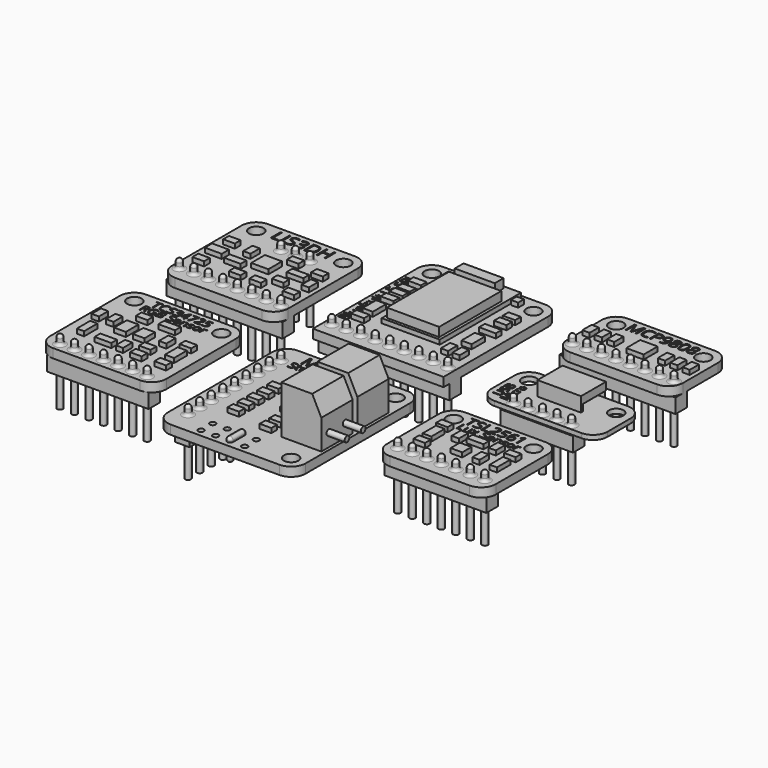
from build123d import *

# Parameters (mm, degrees)
F0_R            = 0.508
F0_R_2          = 1.27
F1_DEPTH        = 1.5875
F2_DEPTH        = 0.79375
F3_W            = 10.16
F3_H            = 17.78
F3_W_2          = 1.27
F3_H_2          = 1.27
F3_W_3          = 2.159
F3_W_4          = 2.921
F3_W_5          = 1.778
F3_H_3          = 2.921
F3_H_4          = 2.032
F3_W_6          = 2.286
F3_H_5          = 2.9464
F4_DEPTH        = 0.79375
F5_W            = 9.144
F5_H            = 13.589
F5_W_2          = 7.0104
F5_H_2          = 1.9304
F6_DEPTH        = 1.5875
F7_W            = 17.78
F7_H            = 2.54
F8_DEPTH        = 2.54
F7_W_2          = 20.32
F7_W_3          = 7.62
F7_R            = 0.508
F7_W_4          = 2.54
F7_H_2          = 22.86
F7_W_5          = 12.7
F7_W_6          = 22.86
F9_DEPTH        = 8.255
F9_DEPTH_BACK   = 3.175
F10_DEPTH       = 0.79375
F11_R           = 0.50799
F11_2_R         = 0.50799
F11_3_R         = 0.50799
F11_4_R         = 0.50799
F11_5_R         = 0.50799
F11_6_R         = 0.50799
F11_7_R         = 0.50799
F13_DEPTH       = 0.762
F13_DEPTH_BACK  = 1.5875
F14_DEPTH       = 1.5875
F15_W           = 6.985
F15_H           = 6.858
F15_R           = 0.508
F16_DEPTH       = 8.382
F17_SIZE2       = 1.5875
F17_SIZE        = 3.175
F18_SIZE2       = 1.5875
F18_SIZE        = 3.175
F19_R           = 0.508
F20_DEPTH       = 3.175
F21_DEPTH       = 1.5875
F21_DEPTH_BACK  = 6.35
F22_R           = 0.50799
F23_W           = 1.27
F23_H           = 2.032
F23_W_2         = 2.032
F23_H_2         = 1.27
F23_W_3         = 2.921
F23_H_3         = 2.921
F24_DEPTH       = 0.79375
F23_W_4         = 7.62
F23_H_4         = 5.4864
F23_W_5         = 2.9464
F23_H_5         = 1.5875
F23_W_6         = 2.9972
F23_H_6         = 2.9972
F23_H_7         = 2.794
F23_H_8         = 2.286
F23_W_7         = 1.5875
F23_W_8         = 1.524
F23_W_9         = 3.048
F23_H_9         = 3.048
F25_DEPTH       = 0.79375
F25_DEPTH_BACK  = 1.74625
F27_DEPTH       = 5.08
F28_TEXT_SIZE   = 3.0305741984
F28_TEXT_SIZE_2 = 2.2091458857
F28_TEXT_SIZE_3 = 2.0715317305
F28_TEXT_SIZE_4 = 2.8646616541
F28_TEXT_SIZE_5 = 2.091610911
F28_TEXT_SIZE_6 = 2.1665037761
F28_TEXT_SIZE_7 = 2.5736521957
F28_TEXT_SIZE_8 = 2.083851119
F28_TEXT_SIZE_9 = 2.7485575399
F29_DEPTH       = 0.254
F30_TEXT_SIZE   = 1.9694693482
F30_TEXT_SIZE_2 = 1.7952644599
F31_DEPTH       = 0.254


# Not quite as in the source:
# - a fillet or chamfer is up to 0.001 mm smaller than in the source, because OpenCascade refuses the exact size
# - Text() gives the source's letters only with a copy of the font that has no kerning and outlines rounded to 1/6400 em; it was checked with that copy


with BuildPart() as f1:
    # F0 (on Top) → F1 (new body)
    with BuildSketch(Plane.XY):
        with BuildLine():
            Line((0, 22.86), (0, 0))
            Line((0, 0), (22.86, 0))
            Line((22.86, 0), (22.86, 22.86))
            ThreePointArc((22.86, 22.86), (22.1160512242, 24.6560512242), (20.32, 25.4))
            Line((20.32, 25.4), (2.54, 25.4))
            ThreePointArc((2.54, 25.4), (0.7439487758, 24.6560512242), (0, 22.86))
        make_face()
        with Locations((1.27, 2.54)):
            Circle(F0_R, mode=Mode.SUBTRACT)
        with Locations((3.81, 2.54)):
            Circle(F0_R, mode=Mode.SUBTRACT)
        with Locations((6.35, 2.54)):
            Circle(F0_R, mode=Mode.SUBTRACT)
        with Locations((8.89, 2.54)):
            Circle(F0_R, mode=Mode.SUBTRACT)
        with Locations((2.54, 22.86)):
            Circle(F0_R_2, mode=Mode.SUBTRACT)
        with Locations((11.43, 2.54)):
            Circle(F0_R, mode=Mode.SUBTRACT)
        with Locations((13.97, 2.54)):
            Circle(F0_R, mode=Mode.SUBTRACT)
        with Locations((16.51, 2.54)):
            Circle(F0_R, mode=Mode.SUBTRACT)
        with Locations((19.05, 2.54)):
            Circle(F0_R, mode=Mode.SUBTRACT)
        with Locations((21.59, 2.54)):
            Circle(F0_R, mode=Mode.SUBTRACT)
        with Locations((20.32, 22.86)):
            Circle(F0_R_2, mode=Mode.SUBTRACT)
    extrude(amount=F1_DEPTH)

    # F3 (on face) → F4 (join)
    with BuildSketch(Plane.XY.offset(1.5875)):
        with Locations((11.43, 16.002)):
            Rectangle(F3_W, F3_H)
        with Locations((5.461, 22.987)):
            Rectangle(F3_W_2, F3_H_2)
        with Locations((17.399, 22.987)):
            Rectangle(F3_W_2, F3_H_2)
        with Locations((19.8755, 18.669)):
            Rectangle(F3_W_3, F3_H_2)
        with Locations((19.8755, 16.764)):
            Rectangle(F3_W_3, F3_H_2)
        with Locations((19.8755, 13.97)):
            Rectangle(F3_W_4, F3_H_2)
        with Locations((19.8755, 10.2235)):
            Rectangle(F3_W_5, F3_H_3)
        with Locations((20.8915, 6.223)):
            Rectangle(F3_W_2, F3_H_4)
        with Locations((18.8595, 6.223)):
            Rectangle(F3_W_2, F3_H_4)
        with Locations((3.3274, 6.223)):
            Rectangle(F3_W_6, F3_H_2)
        with Locations((3.3274, 9.2964)):
            Rectangle(F3_W_5, F3_H_5)
        with Locations((3.3274, 12.7)):
            Rectangle(F3_W_6, F3_H_2)
        with Locations((3.3274, 18.669)):
            Rectangle(F3_W_6, F3_H_2)
        with Locations((3.3274, 16.256)):
            Rectangle(F3_W_6, F3_H_2)
        with Locations((3.3274, 14.605)):
            Rectangle(F3_W_6, F3_H_2)
    extrude(amount=F4_DEPTH)

    # F5 (on face) → F6 (join)
    with BuildSketch(Plane.XY.offset(2.38125)):
        with Locations((11.43, 14.4145)):
            Rectangle(F5_W, F5_H)
        with Locations((10.3632, 23.4188)):
            Rectangle(F5_W_2, F5_H_2)
    extrude(amount=F6_DEPTH)

    # F7 (on face) → F8, piece 5 (join)
    with BuildSketch(Plane(origin=(0, 0, 0), x_dir=(1, 0, 0), z_dir=(0, 0, -1))):
        with Locations((11.43, -2.54)):
            Rectangle(F7_W_6, F7_H)
        with Locations((1.27, -2.54)):
            Circle(F7_R, mode=Mode.SUBTRACT)
        with Locations((3.81, -2.54)):
            Circle(F7_R, mode=Mode.SUBTRACT)
        with Locations((6.35, -2.54)):
            Circle(F7_R, mode=Mode.SUBTRACT)
        with Locations((8.89, -2.54)):
            Circle(F7_R, mode=Mode.SUBTRACT)
        with Locations((11.43, -2.54)):
            Circle(F7_R, mode=Mode.SUBTRACT)
        with Locations((13.97, -2.54)):
            Circle(F7_R, mode=Mode.SUBTRACT)
        with Locations((16.51, -2.54)):
            Circle(F7_R, mode=Mode.SUBTRACT)
        with Locations((19.05, -2.54)):
            Circle(F7_R, mode=Mode.SUBTRACT)
        with Locations((21.59, -2.54)):
            Circle(F7_R, mode=Mode.SUBTRACT)
    extrude(amount=F8_DEPTH)

    # F0 (on Top) → F9 (join, two sides)
    with BuildSketch(Plane.XY) as f9_sk:
        with Locations((1.27, 2.54)):
            Circle(F0_R)
        with Locations((3.81, 2.54)):
            Circle(F0_R)
        with Locations((6.35, 2.54)):
            Circle(F0_R)
        with Locations((8.89, 2.54)):
            Circle(F0_R)
        with Locations((11.43, 2.54)):
            Circle(F0_R)
        with Locations((13.97, 2.54)):
            Circle(F0_R)
        with Locations((16.51, 2.54)):
            Circle(F0_R)
        with Locations((19.05, 2.54)):
            Circle(F0_R)
        with Locations((21.59, 2.54)):
            Circle(F0_R)
    extrude(amount=-F9_DEPTH)
    extrude(f9_sk.sketch, amount=F9_DEPTH_BACK)

    # F11 (radius 0.508 in the source; OpenCascade refuses exactly that, so slightly less here)
    f11_edges = [f1.edges().sort_by_distance(p)[0] for p in [
        (0.762, 2.54, 1.5875),
        (1.778, 2.54, 2.38125),
        (0.762, 2.54, 3.175),
        (3.302, 2.54, 1.5875),
        (4.318, 2.54, 2.38125),
        (3.302, 2.54, 3.175),
        (5.842, 2.54, 1.5875),
        (6.858, 2.54, 2.38125),
        (5.842, 2.54, 3.175),
        (8.382, 2.54, 1.5875),
        (9.398, 2.54, 2.38125),
        (8.382, 2.54, 3.175),
        (10.922, 2.54, 1.5875),
        (11.938, 2.54, 2.38125),
        (10.922, 2.54, 3.175),
        (13.462, 2.54, 1.5875),
        (14.478, 2.54, 2.38125),
        (13.462, 2.54, 3.175),
        (16.002, 2.54, 1.5875),
        (17.018, 2.54, 2.38125),
        (16.002, 2.54, 3.175),
        (18.542, 2.54, 1.5875),
        (19.558, 2.54, 2.38125),
        (18.542, 2.54, 3.175),
        (21.082, 2.54, 1.5875),
        (22.098, 2.54, 2.38125),
        (21.082, 2.54, 3.175),
    ]]
    fillet(f11_edges, radius=F11_R)


with BuildPart() as f1b:
    # F0 (on Top) → F1, piece 2 (new body)
    with BuildSketch(Plane.XY):
        with BuildLine():
            Line((-24.13, 0), (-8.89, 0))
            ThreePointArc((-8.89, 0), (-7.0939487758, 0.7439487758), (-6.35, 2.54))
            Line((-6.35, 2.54), (-6.35, 17.78))
            ThreePointArc((-6.35, 17.78), (-7.0939487758, 19.5760512242), (-8.89, 20.32))
            Line((-8.89, 20.32), (-24.13, 20.32))
            ThreePointArc((-24.13, 20.32), (-25.9260512242, 19.5760512242), (-26.67, 17.78))
            Line((-26.67, 17.78), (-26.67, 2.54))
            ThreePointArc((-26.67, 2.54), (-25.9260512242, 0.7439487758), (-24.13, 0))
        make_face()
        with Locations((-25.4, 2.54)):
            Circle(F0_R, mode=Mode.SUBTRACT)
        with Locations((-22.86, 2.54)):
            Circle(F0_R, mode=Mode.SUBTRACT)
        with Locations((-20.32, 2.54)):
            Circle(F0_R, mode=Mode.SUBTRACT)
        with Locations((-17.78, 2.54)):
            Circle(F0_R, mode=Mode.SUBTRACT)
        with Locations((-15.24, 2.54)):
            Circle(F0_R, mode=Mode.SUBTRACT)
        with Locations((-12.7, 2.54)):
            Circle(F0_R, mode=Mode.SUBTRACT)
        with Locations((-10.16, 2.54)):
            Circle(F0_R, mode=Mode.SUBTRACT)
        with Locations((-7.62, 2.54)):
            Circle(F0_R, mode=Mode.SUBTRACT)
        with Locations((-17.78, 15.24)):
            Circle(F0_R, mode=Mode.SUBTRACT)
        with Locations((-24.13, 17.78)):
            Circle(F0_R_2, mode=Mode.SUBTRACT)
        with Locations((-15.24, 15.24)):
            Circle(F0_R, mode=Mode.SUBTRACT)
        with Locations((-12.7, 15.24)):
            Circle(F0_R, mode=Mode.SUBTRACT)
        with Locations((-8.89, 17.78)):
            Circle(F0_R_2, mode=Mode.SUBTRACT)
    extrude(amount=F1_DEPTH)

    # F7 (on face) → F8, piece 2 (join)
    with BuildSketch(Plane(origin=(0, 0, 0), x_dir=(1, 0, 0), z_dir=(0, 0, -1))):
        with Locations((-16.51, -2.54)):
            Rectangle(F7_W_2, F7_H)
        with Locations((-15.24, -15.24)):
            Rectangle(F7_W_3, F7_H)
        with Locations((-15.24, -15.24)):
            Circle(F7_R, mode=Mode.SUBTRACT)
        with Locations((-15.24, -15.24)):
            Circle(F7_R)
    extrude(amount=F8_DEPTH)

    # F0 (on Top) → F9, piece 2 (join, two sides)
    with BuildSketch(Plane.XY) as f9_2_sk:
        with Locations((-25.4, 2.54)):
            Circle(F0_R)
        with Locations((-22.86, 2.54)):
            Circle(F0_R)
        with Locations((-20.32, 2.54)):
            Circle(F0_R)
        with Locations((-17.78, 2.54)):
            Circle(F0_R)
        with Locations((-15.24, 2.54)):
            Circle(F0_R)
        with Locations((-12.7, 2.54)):
            Circle(F0_R)
        with Locations((-10.16, 2.54)):
            Circle(F0_R)
        with Locations((-7.62, 2.54)):
            Circle(F0_R)
        with Locations((-12.7, 15.24)):
            Circle(F0_R)
        with Locations((-15.24, 15.24)):
            Circle(F0_R)
        with Locations((-17.78, 15.24)):
            Circle(F0_R)
    extrude(amount=-F9_DEPTH)
    extrude(f9_2_sk.sketch, amount=F9_DEPTH_BACK)

    # F11#2 (radius 0.508 in the source; OpenCascade refuses exactly that, so slightly less here)
    f11_2_edges = [f1b.edges().sort_by_distance(p)[0] for p in [
        (-25.908, 2.54, 1.5875),
        (-24.892, 2.54, 2.38125),
        (-25.908, 2.54, 3.175),
        (-23.368, 2.54, 1.5875),
        (-22.352, 2.54, 2.38125),
        (-23.368, 2.54, 3.175),
        (-18.288, 2.54, 1.5875),
        (-17.272, 2.54, 2.38125),
        (-18.288, 2.54, 3.175),
        (-20.828, 2.54, 1.5875),
        (-19.812, 2.54, 2.38125),
        (-20.828, 2.54, 3.175),
        (-15.748, 2.54, 1.5875),
        (-14.732, 2.54, 2.38125),
        (-15.748, 2.54, 3.175),
        (-13.208, 2.54, 1.5875),
        (-12.192, 2.54, 2.38125),
        (-13.208, 2.54, 3.175),
        (-10.668, 2.54, 1.5875),
        (-9.652, 2.54, 2.38125),
        (-10.668, 2.54, 3.175),
        (-8.128, 2.54, 1.5875),
        (-7.112, 2.54, 2.38125),
        (-8.128, 2.54, 3.175),
        (-13.208, 15.24, 1.5875),
        (-12.192, 15.24, 2.38125),
        (-13.208, 15.24, 3.175),
        (-15.748, 15.24, 1.5875),
        (-14.732, 15.24, 2.38125),
        (-15.748, 15.24, 3.175),
        (-18.288, 15.24, 1.5875),
        (-17.272, 15.24, 2.38125),
        (-18.288, 15.24, 3.175),
    ]]
    fillet(f11_2_edges, radius=F11_2_R)

    # F23 (on face) → F24, piece 3 (join)
    with BuildSketch(Plane.XY.offset(1.5875)):
        with Locations((-24.0792, 9.11225)):
            Rectangle(F23_W_5, F23_H_5)
        with Locations((-24.13, 12.446)):
            Rectangle(F23_W_2, F23_H_2)
        with Locations((-20.193, 11.811)):
            Rectangle(F23_W, F23_H)
        with Locations((-20.193, 8.255)):
            Rectangle(F23_W_3, F23_H_2)
        with Locations((-16.2814, 10.2362)):
            Rectangle(F23_W_6, F23_H_6)
        with Locations((-13.589, 13.208)):
            Rectangle(F23_W_2, F23_H_2)
        with Locations((-10.8585, 10.287)):
            Rectangle(F23_W_3, F23_H_2)
        with Locations((-11.684, 7.5184)):
            Rectangle(F23_W_2, F23_H_2)
        with Locations((-7.747, 9.017)):
            Rectangle(F23_W, F23_H)
        with Locations((-8.636, 12.319)):
            Rectangle(F23_W_2, F23_H_2)
        with Locations((-8.255, 5.588)):
            Rectangle(F23_W_2, F23_H_2)
        with Locations((-14.0716, 5.588)):
            Rectangle(F23_W_2, F23_H_2)
        with Locations((-17.653, 5.588)):
            Rectangle(F23_W_2, F23_H_2)
        with Locations((-24.13, 5.715)):
            Rectangle(F23_W_2, F23_H_2)
    extrude(amount=F24_DEPTH)


with BuildPart() as f1c:
    # F0 (on Top) → F1, piece 3 (new body)
    with BuildSketch(Plane.XY):
        with BuildLine():
            ThreePointArc((-6.35, -8.89), (-7.0939487758, -7.0939487758), (-8.89, -6.35))
            Line((-8.89, -6.35), (-24.13, -6.35))
            ThreePointArc((-24.13, -6.35), (-25.9260512242, -7.0939487758), (-26.67, -8.89))
            Line((-26.67, -8.89), (-26.67, -24.13))
            ThreePointArc((-26.67, -24.13), (-25.9260512242, -25.9260512242), (-24.13, -26.67))
            Line((-24.13, -26.67), (-8.89, -26.67))
            ThreePointArc((-8.89, -26.67), (-7.0939487758, -25.9260512242), (-6.35, -24.13))
            Line((-6.35, -24.13), (-6.35, -8.89))
        make_face()
        with Locations((-24.13, -25.146)):
            Circle(F0_R, mode=Mode.SUBTRACT)
        with Locations((-21.59, -25.146)):
            Circle(F0_R, mode=Mode.SUBTRACT)
        with Locations((-19.05, -25.146)):
            Circle(F0_R, mode=Mode.SUBTRACT)
        with Locations((-16.51, -25.146)):
            Circle(F0_R, mode=Mode.SUBTRACT)
        with Locations((-13.97, -25.146)):
            Circle(F0_R, mode=Mode.SUBTRACT)
        with Locations((-11.43, -25.146)):
            Circle(F0_R, mode=Mode.SUBTRACT)
        with Locations((-8.89, -25.146)):
            Circle(F0_R, mode=Mode.SUBTRACT)
        with Locations((-24.13, -8.89)):
            Circle(F0_R_2, mode=Mode.SUBTRACT)
        with Locations((-8.89, -8.89)):
            Circle(F0_R_2, mode=Mode.SUBTRACT)
    extrude(amount=F1_DEPTH)

    # F7 (on face) → F8 (join)
    with BuildSketch(Plane(origin=(0, 0, 0), x_dir=(1, 0, 0), z_dir=(0, 0, -1))):
        with Locations((-16.51, 25.146)):
            Rectangle(F7_W, F7_H)
    extrude(amount=F8_DEPTH)

    # F0 (on Top) → F9, piece 3 (join, two sides)
    with BuildSketch(Plane.XY) as f9_3_sk:
        with Locations((-24.13, -25.146)):
            Circle(F0_R)
        with Locations((-21.59, -25.146)):
            Circle(F0_R)
        with Locations((-19.05, -25.146)):
            Circle(F0_R)
        with Locations((-16.51, -25.146)):
            Circle(F0_R)
        with Locations((-13.97, -25.146)):
            Circle(F0_R)
        with Locations((-11.43, -25.146)):
            Circle(F0_R)
        with Locations((-8.89, -25.146)):
            Circle(F0_R)
    extrude(amount=-F9_DEPTH)
    extrude(f9_3_sk.sketch, amount=F9_DEPTH_BACK)

    # F11#3 (radius 0.508 in the source; OpenCascade refuses exactly that, so slightly less here)
    f11_3_edges = [f1c.edges().sort_by_distance(p)[0] for p in [
        (-9.398, -25.146, 1.5875),
        (-8.382, -25.146, 2.38125),
        (-9.398, -25.146, 3.175),
        (-11.938, -25.146, 1.5875),
        (-10.922, -25.146, 2.38125),
        (-11.938, -25.146, 3.175),
        (-14.478, -25.146, 1.5875),
        (-13.462, -25.146, 2.38125),
        (-14.478, -25.146, 3.175),
        (-17.018, -25.146, 1.5875),
        (-16.002, -25.146, 2.38125),
        (-17.018, -25.146, 3.175),
        (-19.558, -25.146, 1.5875),
        (-18.542, -25.146, 2.38125),
        (-19.558, -25.146, 3.175),
        (-22.098, -25.146, 1.5875),
        (-21.082, -25.146, 2.38125),
        (-22.098, -25.146, 3.175),
        (-24.638, -25.146, 1.5875),
        (-23.622, -25.146, 2.38125),
        (-24.638, -25.146, 3.175),
    ]]
    fillet(f11_3_edges, radius=F11_3_R)

    # F23 (on face) → F24, piece 4 (join)
    with BuildSketch(Plane.XY.offset(1.5875)):
        with Locations((-24.765, -15.621)):
            Rectangle(F23_W, F23_H)
        with Locations((-22.225, -15.621)):
            Rectangle(F23_W, F23_H)
        with Locations((-19.304, -12.7)):
            Rectangle(F23_W_2, F23_H_2)
        with Locations((-19.431, -16.51)):
            Rectangle(F23_W_2, F23_H_7)
        with Locations((-16.256, -16.637)):
            Rectangle(F23_W_2, F23_H_8)
        with Locations((-14.9225, -12.7)):
            Rectangle(F23_W_3, F23_H_2)
        with Locations((-12.573, -16.129)):
            Rectangle(F23_W, F23_H)
        with Locations((-9.398, -15.494)):
            Rectangle(F23_W_2, F23_H_2)
        with Locations((-9.23925, -18.415)):
            Rectangle(F23_W_7, F23_H_7)
        with Locations((-13.208, -21.59)):
            Rectangle(F23_W_2, F23_H_2)
        with Locations((-13.462, -19.304)):
            Rectangle(F23_W_2, F23_H_2)
        with Locations((-16.383, -20.828)):
            Rectangle(F23_W, F23_H)
        with Locations((-19.3675, -21.082)):
            Rectangle(F23_W_3, F23_H_2)
        with Locations((-23.622, -19.8501)):
            Rectangle(F23_W, F23_H_3)
        with Locations((-8.9408, -21.59)):
            Rectangle(F23_W_2, F23_H_2)
    extrude(amount=F24_DEPTH)


with BuildPart() as f1d:
    # F0 (on Top) → F1, piece 4 (new body)
    with BuildSketch(Plane.XY):
        with BuildLine():
            Line((21.59, -6.35), (2.54, -6.35))
            ThreePointArc((2.54, -6.35), (0.7439487758, -7.0939487758), (0, -8.89))
            Line((0, -8.89), (0, -31.75))
            ThreePointArc((0, -31.75), (0.7439487758, -33.5460512242), (2.54, -34.29))
            Line((2.54, -34.29), (21.59, -34.29))
            ThreePointArc((21.59, -34.29), (23.3860512242, -33.5460512242), (24.13, -31.75))
            Line((24.13, -31.75), (24.13, -8.89))
            ThreePointArc((24.13, -8.89), (23.3860512242, -7.0939487758), (21.59, -6.35))
        make_face()
        with Locations((2.54, -30.48)):
            Circle(F0_R, mode=Mode.SUBTRACT)
        with Locations((6.858, -33.02)):
            Circle(F0_R, mode=Mode.SUBTRACT)
        with Locations((9.398, -33.02)):
            Circle(F0_R, mode=Mode.SUBTRACT)
        with Locations((6.858, -30.48)):
            Circle(F0_R, mode=Mode.SUBTRACT)
        with Locations((9.398, -30.48)):
            Circle(F0_R, mode=Mode.SUBTRACT)
        with Locations((2.54, -27.94)):
            Circle(F0_R, mode=Mode.SUBTRACT)
        with Locations((2.54, -25.4)):
            Circle(F0_R, mode=Mode.SUBTRACT)
        with Locations((2.54, -22.86)):
            Circle(F0_R, mode=Mode.SUBTRACT)
        with Locations((2.54, -20.32)):
            Circle(F0_R, mode=Mode.SUBTRACT)
        with Locations((2.54, -17.78)):
            Circle(F0_R, mode=Mode.SUBTRACT)
        with Locations((2.54, -15.24)):
            Circle(F0_R, mode=Mode.SUBTRACT)
        with Locations((2.54, -12.7)):
            Circle(F0_R, mode=Mode.SUBTRACT)
        with Locations((2.54, -10.16)):
            Circle(F0_R, mode=Mode.SUBTRACT)
        with Locations((11.938, -33.02)):
            Circle(F0_R, mode=Mode.SUBTRACT)
        with Locations((14.478, -33.02)):
            Circle(F0_R, mode=Mode.SUBTRACT)
        with Locations((11.938, -30.48)):
            Circle(F0_R, mode=Mode.SUBTRACT)
        with Locations((14.478, -30.48)):
            Circle(F0_R, mode=Mode.SUBTRACT)
        with Locations((21.59, -31.75)):
            Circle(F0_R_2, mode=Mode.SUBTRACT)
        with Locations((20.066, -26.035)):
            Circle(F0_R, mode=Mode.SUBTRACT)
        with Locations((20.066, -22.479)):
            Circle(F0_R, mode=Mode.SUBTRACT)
        with Locations((20.066, -18.161)):
            Circle(F0_R, mode=Mode.SUBTRACT)
        with Locations((20.066, -14.605)):
            Circle(F0_R, mode=Mode.SUBTRACT)
        with Locations((21.59, -8.89)):
            Circle(F0_R_2, mode=Mode.SUBTRACT)
    extrude(amount=F1_DEPTH)

    # F7 (on face) → F8, piece 3 (join)
    with BuildSketch(Plane(origin=(0, 0, 0), x_dir=(1, 0, 0), z_dir=(0, 0, -1))):
        with Locations((2.54, 20.32)):
            Rectangle(F7_W_4, F7_H_2)
    extrude(amount=F8_DEPTH)

    # F0 (on Top) → F9, piece 4 (join, two sides)
    with BuildSketch(Plane.XY) as f9_4_sk:
        with Locations((2.54, -30.48)):
            Circle(F0_R)
        with Locations((2.54, -27.94)):
            Circle(F0_R)
        with Locations((2.54, -25.4)):
            Circle(F0_R)
        with Locations((2.54, -22.86)):
            Circle(F0_R)
        with Locations((2.54, -20.32)):
            Circle(F0_R)
        with Locations((2.54, -17.78)):
            Circle(F0_R)
        with Locations((2.54, -15.24)):
            Circle(F0_R)
        with Locations((2.54, -12.7)):
            Circle(F0_R)
        with Locations((2.54, -10.16)):
            Circle(F0_R)
    extrude(amount=-F9_DEPTH)
    extrude(f9_4_sk.sketch, amount=F9_DEPTH_BACK)

    # F11#4 (radius 0.508 in the source; OpenCascade refuses exactly that, so slightly less here)
    f11_4_edges = [f1d.edges().sort_by_distance(p)[0] for p in [
        (2.032, -17.78, 1.5875),
        (3.048, -17.78, 2.38125),
        (2.032, -17.78, 3.175),
        (2.032, -15.24, 1.5875),
        (3.048, -15.24, 2.38125),
        (2.032, -15.24, 3.175),
        (2.032, -12.7, 1.5875),
        (3.048, -12.7, 2.38125),
        (2.032, -12.7, 3.175),
        (2.032, -10.16, 1.5875),
        (3.048, -10.16, 2.38125),
        (2.032, -10.16, 3.175),
        (2.032, -20.32, 1.5875),
        (3.048, -20.32, 2.38125),
        (2.032, -20.32, 3.175),
        (2.032, -22.86, 1.5875),
        (3.048, -22.86, 2.38125),
        (2.032, -22.86, 3.175),
        (2.032, -25.4, 1.5875),
        (3.048, -25.4, 2.38125),
        (2.032, -25.4, 3.175),
        (2.032, -27.94, 1.5875),
        (3.048, -27.94, 2.38125),
        (2.032, -27.94, 3.175),
        (2.032, -30.48, 1.5875),
        (3.048, -30.48, 2.38125),
        (2.032, -30.48, 3.175),
    ]]
    fillet(f11_4_edges, radius=F11_4_R)

    # F12 (on face) → F13 (join, two sides)
    with BuildSketch(Plane.XY.offset(1.5875)) as f13_sk:
        with BuildLine():
            ThreePointArc((12.446, -30.48), (11.938, -30.988), (11.43, -30.48))
            Line((11.43, -30.48), (11.43, -33.02))
            ThreePointArc((11.43, -33.02), (11.938, -32.512), (12.446, -33.02))
            Line((12.446, -33.02), (12.446, -30.48))
        make_face()
        with BuildLine():
            ThreePointArc((12.446, -30.48), (11.938, -29.972), (11.43, -30.48))
            ThreePointArc((11.43, -30.48), (11.938, -30.988), (12.446, -30.48))
        make_face()
        with BuildLine():
            ThreePointArc((12.446, -33.02), (11.938, -32.512), (11.43, -33.02))
            ThreePointArc((11.43, -33.02), (11.938, -33.528), (12.446, -33.02))
        make_face()
    extrude(amount=F13_DEPTH)
    extrude(f13_sk.sketch, amount=-F13_DEPTH_BACK)

    # F0 (on Top) → F14 (join)
    with BuildSketch(Plane.XY):
        with Locations((11.938, -33.02)):
            Circle(F0_R)
        with Locations((11.938, -30.48)):
            Circle(F0_R)
    extrude(amount=-F14_DEPTH)

    # F15 (on face) → F16 (join)
    with BuildSketch(Plane.XY.offset(1.5875)):
        with Locations((20.1295, -16.383)):
            Rectangle(F15_W, F15_H)
        with Locations((20.066, -18.161)):
            Circle(F15_R, mode=Mode.SUBTRACT)
        with Locations((20.066, -14.605)):
            Circle(F15_R, mode=Mode.SUBTRACT)
        with Locations((20.1295, -24.257)):
            Rectangle(F15_W, F15_H)
        with Locations((20.066, -26.035)):
            Circle(F15_R, mode=Mode.SUBTRACT)
        with Locations((20.066, -22.479)):
            Circle(F15_R, mode=Mode.SUBTRACT)
        with Locations((20.066, -26.035)):
            Circle(F15_R)
        with Locations((20.066, -22.479)):
            Circle(F15_R)
        with Locations((20.066, -14.605)):
            Circle(F15_R)
        with Locations((20.066, -18.161)):
            Circle(F15_R)
    extrude(amount=F16_DEPTH)

    # F17
    f17_edges = [f1d.edges().sort_by_distance(p)[0] for p in [
        (23.622, -24.257, 9.9695),
    ]]
    f17_side = f1d.faces().sort_by_distance((23.622, -24.257, 5.7785))[0]
    chamfer(f17_edges, length=F17_SIZE, length2=F17_SIZE2, reference=f17_side)

    # F18
    f18_edges = [f1d.edges().sort_by_distance(p)[0] for p in [
        (23.622, -16.383, 9.9695),
    ]]
    f18_side = f1d.faces().sort_by_distance((23.622, -16.383, 5.7785))[0]
    chamfer(f18_edges, length=F18_SIZE, length2=F18_SIZE2, reference=f18_side)

    # F19 (on face) → F20 (join)
    with BuildSketch(Plane.YZ.offset(23.622)):
        with Locations((-26.035, 3.8735)):
            Circle(F19_R)
        with Locations((-22.479, 3.8735)):
            Circle(F19_R)
    extrude(amount=F20_DEPTH)

    # F0 (on Top) → F21 (join, two sides)
    with BuildSketch(Plane.XY) as f21_sk:
        with Locations((20.066, -26.035)):
            Circle(F0_R)
        with Locations((20.066, -22.479)):
            Circle(F0_R)
    extrude(amount=-F21_DEPTH)
    extrude(f21_sk.sketch, amount=F21_DEPTH_BACK)

    # F22 (radius 0.508 in the source; OpenCascade refuses exactly that, so slightly less here)
    f22_edges = [f1d.edges().sort_by_distance(p)[0] for p in [
        (12.446, -33.02, -0.79375),
        (11.43, -33.02, 0),
        (11.43, -33.02, -1.5875),
        (12.446, -30.48, -0.79375),
        (11.43, -30.48, 0),
        (11.43, -30.48, -1.5875),
        (20.574, -22.479, -0.79375),
        (19.558, -22.479, 0),
        (19.558, -22.479, -1.5875),
        (20.574, -26.035, -0.79375),
        (19.558, -26.035, 0),
        (19.558, -26.035, -1.5875),
        (11.43, -31.75, 2.3495),
        (11.938, -33.528, 2.3495),
        (12.446, -31.75, 2.3495),
        (11.938, -29.972, 2.3495),
    ]]
    fillet(f22_edges, radius=F22_R)

    # F23 (on face) → F24 (join)
    with BuildSketch(Plane.XY.offset(1.5875)):
        with Locations((8.5598, -14.605)):
            Rectangle(F23_W, F23_H)
        with Locations((7.3914, -17.399)):
            Rectangle(F23_W_2, F23_H_2)
        with Locations((7.3914, -19.558)):
            Rectangle(F23_W_2, F23_H_2)
        with Locations((7.3914, -21.717)):
            Rectangle(F23_W_2, F23_H_2)
        with Locations((7.3914, -23.876)):
            Rectangle(F23_W_2, F23_H_2)
        with Locations((7.3914, -26.035)):
            Rectangle(F23_W_2, F23_H_2)
        with Locations((13.2969, -20.5105)):
            Rectangle(F23_W_3, F23_H_3)
        with Locations((13.8684, -24.9936)):
            Rectangle(F23_W_2, F23_H_2)
        with Locations((13.8684, -27.0637)):
            Rectangle(F23_W_2, F23_H_2)
        with Locations((12.065, -15.494)):
            Rectangle(F23_W, F23_H)
        with Locations((14.2494, -15.494)):
            Rectangle(F23_W, F23_H)
    extrude(amount=F24_DEPTH)


with BuildPart() as f1e:
    # F0 (on Top) → F1, piece 5 (new body)
    with BuildSketch(Plane.XY):
        with BuildLine():
            Line((45.72, -6.35), (31.75, -6.35))
            ThreePointArc((31.75, -6.35), (29.9539487758, -7.0939487758), (29.21, -8.89))
            Line((29.21, -8.89), (29.21, -20.32))
            ThreePointArc((29.21, -20.32), (29.9539487758, -22.1160512242), (31.75, -22.86))
            Line((31.75, -22.86), (45.72, -22.86))
            ThreePointArc((45.72, -22.86), (47.5160512242, -22.1160512242), (48.26, -20.32))
            Line((48.26, -20.32), (48.26, -8.89))
            ThreePointArc((48.26, -8.89), (47.5160512242, -7.0939487758), (45.72, -6.35))
        make_face()
        with Locations((31.115, -20.32)):
            Circle(F0_R, mode=Mode.SUBTRACT)
        with Locations((33.655, -20.32)):
            Circle(F0_R, mode=Mode.SUBTRACT)
        with Locations((36.195, -20.32)):
            Circle(F0_R, mode=Mode.SUBTRACT)
        with Locations((38.735, -20.32)):
            Circle(F0_R, mode=Mode.SUBTRACT)
        with Locations((41.275, -20.32)):
            Circle(F0_R, mode=Mode.SUBTRACT)
        with Locations((43.815, -20.32)):
            Circle(F0_R, mode=Mode.SUBTRACT)
        with Locations((46.355, -20.32)):
            Circle(F0_R, mode=Mode.SUBTRACT)
        with Locations((31.75, -8.89)):
            Circle(F0_R_2, mode=Mode.SUBTRACT)
        with Locations((45.72, -8.89)):
            Circle(F0_R_2, mode=Mode.SUBTRACT)
    extrude(amount=F1_DEPTH)

    # F7 (on face) → F8, piece 6 (join)
    with BuildSketch(Plane(origin=(0, 0, 0), x_dir=(1, 0, 0), z_dir=(0, 0, -1))):
        with Locations((38.735, 20.32)):
            Rectangle(F7_W, F7_H)
    extrude(amount=F8_DEPTH)

    # F0 (on Top) → F9, piece 6 (join, two sides)
    with BuildSketch(Plane.XY) as f9_6_sk:
        with Locations((46.355, -20.32)):
            Circle(F0_R)
        with Locations((43.815, -20.32)):
            Circle(F0_R)
        with Locations((41.275, -20.32)):
            Circle(F0_R)
        with Locations((38.735, -20.32)):
            Circle(F0_R)
        with Locations((36.195, -20.32)):
            Circle(F0_R)
        with Locations((33.655, -20.32)):
            Circle(F0_R)
        with Locations((31.115, -20.32)):
            Circle(F0_R)
    extrude(amount=-F9_DEPTH)
    extrude(f9_6_sk.sketch, amount=F9_DEPTH_BACK)

    # F11#5 (radius 0.508 in the source; OpenCascade refuses exactly that, so slightly less here)
    f11_5_edges = [f1e.edges().sort_by_distance(p)[0] for p in [
        (38.227, -20.32, 1.5875),
        (39.243, -20.32, 2.38125),
        (38.227, -20.32, 3.175),
        (35.687, -20.32, 1.5875),
        (36.703, -20.32, 2.38125),
        (35.687, -20.32, 3.175),
        (33.147, -20.32, 1.5875),
        (34.163, -20.32, 2.38125),
        (33.147, -20.32, 3.175),
        (40.767, -20.32, 1.5875),
        (41.783, -20.32, 2.38125),
        (40.767, -20.32, 3.175),
        (43.307, -20.32, 1.5875),
        (44.323, -20.32, 2.38125),
        (43.307, -20.32, 3.175),
        (45.847, -20.32, 1.5875),
        (46.863, -20.32, 2.38125),
        (45.847, -20.32, 3.175),
        (30.607, -20.32, 1.5875),
        (31.623, -20.32, 2.38125),
        (30.607, -20.32, 3.175),
    ]]
    fillet(f11_5_edges, radius=F11_5_R)

    # F23 (on face) → F24, piece 5 (join)
    with BuildSketch(Plane.XY.offset(1.5875)):
        with Locations((32.512, -11.811)):
            Rectangle(F23_W_2, F23_H_2)
        with Locations((32.766, -14.5415)):
            Rectangle(F23_W_8, F23_H_3)
        with Locations((33.02, -17.399)):
            Rectangle(F23_W_2, F23_H_2)
        with Locations((36.195, -13.081)):
            Rectangle(F23_W, F23_H)
        with Locations((39.0525, -12.7)):
            Rectangle(F23_W_3, F23_H_2)
        with Locations((38.735, -16.002)):
            Rectangle(F23_W_2, F23_H)
        with Locations((42.3418, -16.256)):
            Rectangle(F23_W, F23_H)
        with Locations((42.3418, -12.7)):
            Rectangle(F23_W, F23_H)
        with Locations((45.339, -12.954)):
            Rectangle(F23_W_2, F23_H_2)
        with Locations((45.593, -16.0655)):
            Rectangle(F23_W, F23_H_3)
    extrude(amount=F24_DEPTH)


with BuildPart() as f1f:
    # F0 (on Top) → F1, piece 6 (new body)
    with BuildSketch(Plane.XY):
        with BuildLine():
            ThreePointArc((29.21, 19.05), (29.9539487758, 17.2539487758), (31.75, 16.51))
            Line((31.75, 16.51), (46.99, 16.51))
            ThreePointArc((46.99, 16.51), (48.7860512242, 17.2539487758), (49.53, 19.05))
            Line((49.53, 19.05), (49.53, 26.67))
            ThreePointArc((49.53, 26.67), (48.7860512242, 28.4660512242), (46.99, 29.21))
            Line((46.99, 29.21), (31.75, 29.21))
            ThreePointArc((31.75, 29.21), (29.9539487758, 28.4660512242), (29.21, 26.67))
            Line((29.21, 26.67), (29.21, 19.05))
        make_face()
        with Locations((30.48, 18.669)):
            Circle(F0_R, mode=Mode.SUBTRACT)
        with Locations((33.02, 18.669)):
            Circle(F0_R, mode=Mode.SUBTRACT)
        with Locations((35.56, 18.669)):
            Circle(F0_R, mode=Mode.SUBTRACT)
        with Locations((38.1, 18.669)):
            Circle(F0_R, mode=Mode.SUBTRACT)
        with Locations((40.64, 18.669)):
            Circle(F0_R, mode=Mode.SUBTRACT)
        with Locations((43.18, 18.669)):
            Circle(F0_R, mode=Mode.SUBTRACT)
        with Locations((45.72, 18.669)):
            Circle(F0_R, mode=Mode.SUBTRACT)
        with Locations((48.26, 18.669)):
            Circle(F0_R, mode=Mode.SUBTRACT)
        with Locations((31.75, 26.67)):
            Circle(F0_R_2, mode=Mode.SUBTRACT)
        with Locations((46.99, 26.67)):
            Circle(F0_R_2, mode=Mode.SUBTRACT)
    extrude(amount=F1_DEPTH)

    # F7 (on face) → F8, piece 7 (join)
    with BuildSketch(Plane(origin=(0, 0, 0), x_dir=(1, 0, 0), z_dir=(0, 0, -1))):
        with Locations((39.37, -18.669)):
            Rectangle(F7_W_2, F7_H)
    extrude(amount=F8_DEPTH)

    # F0 (on Top) → F9, piece 7 (join, two sides)
    with BuildSketch(Plane.XY) as f9_7_sk:
        with Locations((48.26, 18.669)):
            Circle(F0_R)
        with Locations((45.72, 18.669)):
            Circle(F0_R)
        with Locations((43.18, 18.669)):
            Circle(F0_R)
        with Locations((40.64, 18.669)):
            Circle(F0_R)
        with Locations((38.1, 18.669)):
            Circle(F0_R)
        with Locations((35.56, 18.669)):
            Circle(F0_R)
        with Locations((33.02, 18.669)):
            Circle(F0_R)
        with Locations((30.48, 18.669)):
            Circle(F0_R)
    extrude(amount=-F9_DEPTH)
    extrude(f9_7_sk.sketch, amount=F9_DEPTH_BACK)

    # F11#6 (radius 0.508 in the source; OpenCascade refuses exactly that, so slightly less here)
    f11_6_edges = [f1f.edges().sort_by_distance(p)[0] for p in [
        (29.972, 18.669, 1.5875),
        (30.988, 18.669, 2.38125),
        (29.972, 18.669, 3.175),
        (32.512, 18.669, 1.5875),
        (33.528, 18.669, 2.38125),
        (32.512, 18.669, 3.175),
        (35.052, 18.669, 1.5875),
        (36.068, 18.669, 2.38125),
        (35.052, 18.669, 3.175),
        (37.592, 18.669, 1.5875),
        (38.608, 18.669, 2.38125),
        (37.592, 18.669, 3.175),
        (40.132, 18.669, 1.5875),
        (41.148, 18.669, 2.38125),
        (40.132, 18.669, 3.175),
        (42.672, 18.669, 1.5875),
        (43.688, 18.669, 2.38125),
        (42.672, 18.669, 3.175),
        (45.212, 18.669, 1.5875),
        (46.228, 18.669, 2.38125),
        (45.212, 18.669, 3.175),
        (47.752, 18.669, 1.5875),
        (48.768, 18.669, 2.38125),
        (47.752, 18.669, 3.175),
    ]]
    fillet(f11_6_edges, radius=F11_6_R)

    # F23 (on face) → F24, piece 6 (join)
    with BuildSketch(Plane.XY.offset(1.5875)):
        with Locations((30.607, 22.479)):
            Rectangle(F23_W, F23_H)
        with Locations((32.766, 22.479)):
            Rectangle(F23_W, F23_H)
        with Locations((34.925, 22.479)):
            Rectangle(F23_W, F23_H)
        with Locations((39.497, 22.606)):
            Rectangle(F23_W_9, F23_H_9)
        with Locations((43.815, 22.479)):
            Rectangle(F23_W, F23_H)
        with Locations((48.133, 22.479)):
            Rectangle(F23_W, F23_H)
        with Locations((45.974, 22.479)):
            Rectangle(F23_W, F23_H)
    extrude(amount=F24_DEPTH)


with BuildPart() as f2:
    # F0 (on Top) → F2 (new body)
    with BuildSketch(Plane.XY):
        with BuildLine():
            ThreePointArc((29.21, 2.54), (29.9539487758, 0.7439487758), (31.75, 0))
            Line((31.75, 0), (46.99, 0))
            ThreePointArc((46.99, 0), (48.7860512242, 0.7439487758), (49.53, 2.54))
            Line((49.53, 2.54), (49.53, 7.62))
            ThreePointArc((49.53, 7.62), (48.7860512242, 9.4160512242), (46.99, 10.16))
            Line((46.99, 10.16), (31.75, 10.16))
            ThreePointArc((31.75, 10.16), (29.9539487758, 9.4160512242), (29.21, 7.62))
            Line((29.21, 7.62), (29.21, 2.54))
        make_face()
        with Locations((34.29, 1.016)):
            Circle(F0_R, mode=Mode.SUBTRACT)
        with Locations((36.83, 1.016)):
            Circle(F0_R, mode=Mode.SUBTRACT)
        with Locations((39.37, 1.016)):
            Circle(F0_R, mode=Mode.SUBTRACT)
        with Locations((41.91, 1.016)):
            Circle(F0_R, mode=Mode.SUBTRACT)
        with Locations((44.45, 1.016)):
            Circle(F0_R, mode=Mode.SUBTRACT)
        with Locations((31.75, 7.62)):
            Circle(F0_R_2, mode=Mode.SUBTRACT)
        with Locations((46.99, 7.62)):
            Circle(F0_R_2, mode=Mode.SUBTRACT)
    extrude(amount=F2_DEPTH)

    # F7 (on face) → F8, piece 4 (join)
    with BuildSketch(Plane(origin=(0, 0, 0), x_dir=(1, 0, 0), z_dir=(0, 0, -1))):
        with Locations((39.37, -1.016)):
            Rectangle(F7_W_5, F7_H)
    extrude(amount=F8_DEPTH)

    # F0 (on Top) → F9, piece 5 (join, two sides)
    with BuildSketch(Plane.XY) as f9_5_sk:
        with Locations((34.29, 1.016)):
            Circle(F0_R)
        with Locations((36.83, 1.016)):
            Circle(F0_R)
        with Locations((39.37, 1.016)):
            Circle(F0_R)
        with Locations((41.91, 1.016)):
            Circle(F0_R)
        with Locations((44.45, 1.016)):
            Circle(F0_R)
    extrude(amount=-F9_DEPTH)
    extrude(f9_5_sk.sketch, amount=F9_DEPTH_BACK)

    # F10 (cut): faces of the model
    f10_faces = [f2.faces().sort_by_distance(p)[0] for p in [
        (34.29, 1.016, 3.175),
        (36.83, 1.016, 3.175),
        (39.37, 1.016, 3.175),
        (41.91, 1.016, 3.175),
        (44.45, 1.016, 3.175),
    ]]
    extrude(f10_faces, amount=-F10_DEPTH, mode=Mode.SUBTRACT)

    # F11#7 (radius 0.508 in the source; OpenCascade refuses exactly that, so slightly less here)
    f11_7_edges = [f2.edges().sort_by_distance(p)[0] for p in [
        (34.798, 1.016, 1.5875),
        (33.782, 1.016, 2.38125),
        (33.782, 1.016, 0.79375),
        (37.338, 1.016, 1.5875),
        (36.322, 1.016, 2.38125),
        (36.322, 1.016, 0.79375),
        (39.878, 1.016, 1.5875),
        (38.862, 1.016, 2.38125),
        (38.862, 1.016, 0.79375),
        (42.418, 1.016, 1.5875),
        (41.402, 1.016, 2.38125),
        (41.402, 1.016, 0.79375),
        (44.958, 1.016, 1.5875),
        (43.942, 1.016, 2.38125),
        (43.942, 1.016, 0.79375),
    ]]
    fillet(f11_7_edges, radius=F11_7_R)



with BuildPart() as f24:
    # F23 (on face) → F24, piece 2 (new body)
    with BuildSketch(Plane.XY.offset(1.5875)):
        with Locations((39.37, 7.4168)):
            Rectangle(F23_W_4, F23_H_4)
    extrude(amount=F24_DEPTH)


with BuildPart() as f2_1:
    add(f2.part)
    # F25 (add, two sides): a face of the model
    f25_faces = [f24.part.faces().sort_by_distance(p)[0] for p in [
        (39.37, 7.4168, 1.5875),
    ]]

    add(f24.part)  # F25 merges F24
    extrude(f25_faces, amount=F25_DEPTH)
    extrude(f25_faces, amount=-F25_DEPTH_BACK)

    # F26 (on face) → F27 (cut)
    with BuildSketch(Plane(origin=(0, 10.16, 0), x_dir=(-1, 0, 0), z_dir=(0, 1, 0))):
        Polygon((-43.18, 1.9719427711), (-43.18, 0.79375), (-41.783, 0.79375), align=None)
        Polygon((-35.56, 0.79375), (-35.56, 1.9719427711), (-36.957, 0.79375), align=None)
        Polygon((-35.9029, 3.07975), (-42.8371, 3.07975), (-42.8371, 2.06375), (-41.783, 1.17475), (-36.957, 1.17475), (-35.9029, 2.06375), align=None)
    extrude(amount=-F27_DEPTH, mode=Mode.SUBTRACT)

    # F30 (on face) → F31 (cut)
    with BuildSketch(Plane.XY.offset(0.79375)):
        with Locations(Location((31.4217679307, 1.5875), (0, 0, 90))):
            Text('USB', F30_TEXT_SIZE, font='Open Sans', text_align=(TextAlign.LEFT, TextAlign.BOTTOM))
        with Locations(Location((32.9683583418, 1.11125), (0, 0, 90))):
            Text('Micro', F30_TEXT_SIZE_2, font='Open Sans', text_align=(TextAlign.LEFT, TextAlign.BOTTOM))
    extrude(amount=-F31_DEPTH, mode=Mode.SUBTRACT)


with BuildPart() as f29_tool:
    # F28 (on face) → F29 (new body)
    with BuildSketch(Plane.XY.offset(1.5875)):
        with Locations((-21.59, 17.3442365772)):
            Text('LIS3DH', F28_TEXT_SIZE, font='Open Sans', text_align=(TextAlign.LEFT, TextAlign.BOTTOM))
        with Locations((-21.59, -8.7343350377)):
            Text('TCS34725', F28_TEXT_SIZE_2, font='Open Sans', text_align=(TextAlign.LEFT, TextAlign.BOTTOM))
        with Locations((-22.225, -10.4798378837)):
            Text('RGB Sensor', F28_TEXT_SIZE_3, font='Open Sans', text_align=(TextAlign.LEFT, TextAlign.BOTTOM))
        with Locations((4.92125, -9.206306391)):
            Text('MAX98306', F28_TEXT_SIZE_4, font='Open Sans', text_align=(TextAlign.LEFT, TextAlign.BOTTOM))
        with Locations((4.1275, -10.9662662469)):
            Text('Stereo Amplifier', F28_TEXT_SIZE_5, font='Open Sans', text_align=(TextAlign.LEFT, TextAlign.BOTTOM))
        with Locations(Location((1.9408827188, 4.7625), (0, 0, 90))):
            Text('Bluefruit LE SPI', F28_TEXT_SIZE_6, font='Open Sans', text_align=(TextAlign.LEFT, TextAlign.BOTTOM))
        with Locations((33.528, -8.9967795809)):
            Text('TSL2561', F28_TEXT_SIZE_7, font='Open Sans', text_align=(TextAlign.LEFT, TextAlign.BOTTOM))
        with Locations((33.528, -10.7511523866)):
            Text('Lux Sensor', F28_TEXT_SIZE_8, font='Open Sans', text_align=(TextAlign.LEFT, TextAlign.BOTTOM))
        with Locations((33.274, 26.4372885713)):
            Text('MCP9808', F28_TEXT_SIZE_9, font='Open Sans', text_align=(TextAlign.LEFT, TextAlign.BOTTOM))
    extrude(amount=-F29_DEPTH)


with BuildPart() as f1_1:
    add(f1.part)

    # F29: cut by f29_tool
    add(f29_tool.part, mode=Mode.SUBTRACT)


with BuildPart() as f1b_1:
    add(f1b.part)

    # F29: cut by f29_tool
    add(f29_tool.part, mode=Mode.SUBTRACT)


with BuildPart() as f1c_1:
    add(f1c.part)

    # F29: cut by f29_tool
    add(f29_tool.part, mode=Mode.SUBTRACT)


with BuildPart() as f1d_1:
    add(f1d.part)

    # F29: cut by f29_tool
    add(f29_tool.part, mode=Mode.SUBTRACT)


with BuildPart() as f1e_1:
    add(f1e.part)

    # F29: cut by f29_tool
    add(f29_tool.part, mode=Mode.SUBTRACT)


with BuildPart() as f1f_1:
    add(f1f.part)

    # F29: cut by f29_tool
    add(f29_tool.part, mode=Mode.SUBTRACT)


solid = Compound([f2_1.part, f1_1.part, f1b_1.part, f1c_1.part, f1d_1.part, f1e_1.part, f1f_1.part])
